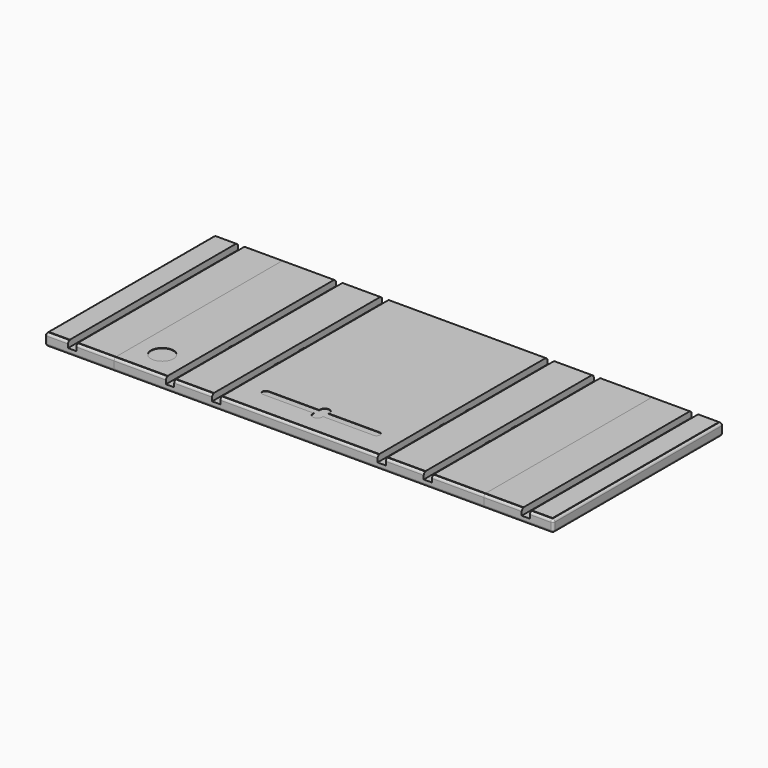
from build123d import *

# Parameters (mm, degrees)
F0_W         = 800
F0_H         = 460
F1_DEPTH     = 25
F2_R         = 5
F3_W         = 18
F3_H         = 13
F4_DEPTH     = 250
F6_DEPTH     = 25
F7_R         = 5
F7_2_R       = 5
F8_W         = 18
F8_H         = 13
F9_DEPTH     = 250
F10_W        = 150
F10_H        = 24
F11_DEPTH    = 30
F13_DEPTH    = 300
F14_R        = 20
F15_T1_DEPTH = 9
F16_R        = 5
F17_W        = 45
F17_H        = 450
F18_DEPTH    = 1
F17_W_2      = 82
F17_W_3      = 340
F19_DEPTH    = 1
F20_W        = 10
F20_H        = 15
F21_DEPTH    = 1
F22_R        = 24.5
F23_DEPTH    = 1


# Not quite as in the source:
# - a fillet or chamfer that OpenCascade refuses, or shapes differently, is made with other operations: its cross-section is extruded or revolved along the edge and cut away or added


with BuildPart() as f1:
    # F0 (on Top) → F1 (new body)
    with BuildSketch(Plane.XY):
        Rectangle(F0_W, F0_H)
    extrude(amount=F1_DEPTH)

    # F2
    f2_edges = [f1.edges().sort_by_distance(p)[0] for p in [
        (0, -230, 25),
        (0, 230, 25),
        (0, 230, 0),
        (0, -230, 0),
    ]]
    fillet(f2_edges, radius=F2_R)

    # F3 (on Front) → F4 (cut, symmetric)
    with BuildSketch(Plane.XZ):
        with Locations((-179, 18.5)):
            Rectangle(F3_W, F3_H)
        with Locations((-279, 18.5)):
            Rectangle(F3_W, F3_H)
        with Locations((179, 18.5)):
            Rectangle(F3_W, F3_H)
        with Locations((279, 18.5)):
            Rectangle(F3_W, F3_H)
    extrude(amount=F4_DEPTH, both=True, mode=Mode.SUBTRACT)

    # F10 (on Right) → F11 (cut, symmetric)
    with BuildSketch(Plane.YZ):
        with Locations((-11.93539612, 0)):
            Rectangle(F10_W, F10_H)
    extrude(amount=F11_DEPTH, both=True, mode=Mode.SUBTRACT)

    # F12 (on Right) → F13 (cut, symmetric)
    with BuildSketch(Plane.YZ):
        Polygon((-61.0856295228, 0), (-52.0856295228, 0), (-52.0856295228, 3), (-50.5856295228, 3), (-50.5856295228, 13), (-62.5856295228, 13), (-62.5856295228, 3), (-61.0856295228, 3), align=None)
        Polygon((6.4143704772, 3), (7.9143704772, 3), (7.9143704772, 0), (16.9143704772, 0), (16.9143704772, 3), (18.4143704772, 3), (18.4143704772, 13), (6.4143704772, 13), align=None)
    extrude(amount=F13_DEPTH, both=True, mode=Mode.SUBTRACT)

    # F14
    f14_edges = [f1.edges().sort_by_distance(p)[0] for p in [
        (30, -86.935396, 6),
        (-30, -86.935396, 6),
        (-30, 63.064604, 6),
        (30, 63.064604, 6),
    ]]
    fillet(f14_edges, radius=F14_R)

    # F15: fillet of radius 5 on 8 edges, made by hand

    # F15_s2 → F15_t1 (cut)
    with BuildSketch(Plane.XY.offset(3)):
        with BuildLine():
            ThreePointArc((-29.9932339999, -67.4555828422), (-31.5022899583, -64.0044123133), (-34.9915424999, -62.5856295228))
            Line((-34.9915424999, -62.5856295228), (-34.9915424999, -62.0856295228))
            Line((-34.9915424999, -62.0856295228), (-30, -62.0856295228))
            Line((-30, -62.0856295228), (-29.5, -62.5856295228))
            ThreePointArc((-29.5, -62.5856295228), (-29.5, -66.93539612), (-29.4934031499, -67.4425781742))
            Line((-29.4934031499, -67.4425781742), (-29.9932339999, -67.4555828422))
        make_face()
        with BuildLine():
            ThreePointArc((-30, -45.5856295228), (-31.4644660941, -49.1211634287), (-35, -50.5856295228))
            Line((-35, -50.5856295228), (-30, -50.5856295228))
            Line((-30, -50.5856295228), (-30, -45.5856295228))
        make_face()
        with BuildLine():
            ThreePointArc((-30, 1.4143704772), (-31.4644660941, 4.9499043831), (-35, 6.4143704772))
            Line((-35, 6.4143704772), (-30, 6.4143704772))
            Line((-30, 6.4143704772), (-30, 1.4143704772))
        make_face()
        with BuildLine():
            ThreePointArc((-30, 23.4143704772), (-31.4644660941, 19.8788365713), (-35, 18.4143704772))
            Line((-35, 18.4143704772), (-30, 18.4143704772))
            Line((-30, 18.4143704772), (-30, 23.4143704772))
        make_face()
        with BuildLine():
            ThreePointArc((29.9932339999, -67.4555828422), (31.5022899583, -64.0044123133), (34.9915424999, -62.5856295228))
            Line((34.9915424999, -62.5856295228), (34.9915424999, -62.0856295228))
            Line((34.9915424999, -62.0856295228), (30, -62.0856295228))
            Line((30, -62.0856295228), (29.5, -62.5856295228))
            ThreePointArc((29.5, -62.5856295228), (29.5, -66.93539612), (29.4934031499, -67.4425781742))
            Line((29.4934031499, -67.4425781742), (29.9932339999, -67.4555828422))
        make_face()
        with BuildLine():
            ThreePointArc((30, -45.5856295228), (31.4644660941, -49.1211634287), (35, -50.5856295228))
            Line((35, -50.5856295228), (30, -50.5856295228))
            Line((30, -50.5856295228), (30, -45.5856295228))
        make_face()
        with BuildLine():
            ThreePointArc((30, 1.4143704772), (31.4644660941, 4.9499043831), (35, 6.4143704772))
            Line((35, 6.4143704772), (30, 6.4143704772))
            Line((30, 6.4143704772), (30, 1.4143704772))
        make_face()
        with BuildLine():
            ThreePointArc((30, 23.4143704772), (31.4644660941, 19.8788365713), (35, 18.4143704772))
            Line((35, 18.4143704772), (30, 18.4143704772))
            Line((30, 18.4143704772), (30, 23.4143704772))
        make_face()
    extrude(amount=F15_T1_DEPTH, mode=Mode.SUBTRACT)

    # F16
    f16_edges = [f1.edges().sort_by_distance(p)[0] for p in [
        (-30, -61.08563, 1.5),
        (-30, -52.08563, 1.5),
        (-30, 7.91437, 1.5),
        (-30, 16.91437, 1.5),
        (30, 16.91437, 1.5),
        (30, 7.91437, 1.5),
        (30, -52.08563, 1.5),
        (30, -61.08563, 1.5),
    ]]
    fillet(f16_edges, radius=F16_R)


with BuildPart() as f6:
    # F5 (on Top) → F6 (new body)
    with BuildSketch(Plane.XY):
        Polygon((-400, -230), (-400, 0), (-400, 230), (-550, 230), (-550, -230), align=None)
    extrude(amount=F6_DEPTH)

    # F7
    f7_edges = [f6.edges().sort_by_distance(p)[0] for p in [
        (-475, 230, 25),
        (-550, 0, 25),
        (-475, -230, 25),
        (-475, -230, 0),
        (-550, 0, 0),
        (-475, 230, 0),
        (-550, -230, 12.5),
        (-550, 230, 12.5),
    ]]
    fillet(f7_edges, radius=F7_R)


with BuildPart() as f6b:
    # F5 (on Top) → F6, piece 2 (new body)
    with BuildSketch(Plane.XY):
        Polygon((400, 0), (400, -230), (550, -230), (550, 230), (400, 230), align=None)
    extrude(amount=F6_DEPTH)

    # F7#2
    f7_2_edges = [f6b.edges().sort_by_distance(p)[0] for p in [
        (475, 230, 0),
        (550, 0, 0),
        (475, -230, 0),
        (475, 230, 25),
        (475, -230, 25),
        (550, 0, 25),
        (550, -230, 12.5),
        (550, 230, 12.5),
    ]]
    fillet(f7_2_edges, radius=F7_2_R)


with BuildPart() as f9_tool:
    # F8 (on Front) → F9 (new body, symmetric)
    with BuildSketch(Plane.XZ):
        with Locations((-491, 18.5)):
            Rectangle(F8_W, F8_H)
        with Locations((491, 18.5)):
            Rectangle(F8_W, F8_H)
    extrude(amount=F9_DEPTH, both=True)


with BuildPart() as f6_1:
    add(f6.part)

    # F9: cut by f9_tool
    add(f9_tool.part, mode=Mode.SUBTRACT)


with BuildPart() as f6b_1:
    add(f6b.part)

    # F9: cut by f9_tool
    add(f9_tool.part, mode=Mode.SUBTRACT)


with BuildPart() as f18:
    # F17 (on face) → F18 (new body)
    with BuildSketch(Plane.XY.offset(25)):
        with Locations((-522.5, 0)):
            Rectangle(F17_W, F17_H)
    extrude(amount=F18_DEPTH)


with BuildPart() as f18b:
    # F17 (on face) → F18, piece 2 (new body)
    with BuildSketch(Plane.XY.offset(25)):
        with Locations((-441, 0)):
            Rectangle(F17_W_2, F17_H)
    extrude(amount=F18_DEPTH)


with BuildPart() as f18c:
    # F17 (on face) → F18, piece 3 (new body)
    with BuildSketch(Plane.XY.offset(25)):
        with Locations((-229, 0)):
            Rectangle(F17_W_2, F17_H)
    extrude(amount=F18_DEPTH)


with BuildPart() as f18d:
    # F17 (on face) → F18, piece 4 (new body)
    with BuildSketch(Plane.XY.offset(25)):
        Rectangle(F17_W_3, F17_H)
    extrude(amount=F18_DEPTH)

    # F20 (on face) → F21 (cut)
    with BuildSketch(Plane.XY.offset(26)):
        with BuildLine():
            ThreePointArc((-120, -162.5), (-127.5, -170), (-120, -177.5))
            Line((-120, -177.5), (-10, -177.5))
            Line((-10, -177.5), (-10, -162.5))
            Line((-10, -162.5), (-120, -162.5))
        make_face()
        with Locations((-5, -170)):
            Rectangle(F20_W, F20_H)
        with BuildLine():
            Line((0, -177.5), (-10, -177.5))
            Line((-10, -177.5), (-10, -180))
            ThreePointArc((-10, -180), (0, -190), (10, -180))
            Line((10, -180), (10, -177.5))
            Line((10, -177.5), (0, -177.5))
        make_face()
        with BuildLine():
            Line((-10, -160), (-10, -162.5))
            Line((-10, -162.5), (0, -162.5))
            Line((0, -162.5), (10, -162.5))
            Line((10, -162.5), (10, -160))
            ThreePointArc((10, -160), (0, -150), (-10, -160))
        make_face()
        with Locations((5, -170)):
            Rectangle(F20_W, F20_H)
        with BuildLine():
            Line((10, -162.5), (10, -177.5))
            Line((10, -177.5), (120, -177.5))
            ThreePointArc((120, -177.5), (127.5, -170), (120, -162.5))
            Line((120, -162.5), (10, -162.5))
        make_face()
    extrude(amount=-F21_DEPTH, mode=Mode.SUBTRACT)


with BuildPart() as f18e:
    # F17 (on face) → F18, piece 5 (new body)
    with BuildSketch(Plane.XY.offset(25)):
        with Locations((229, 0)):
            Rectangle(F17_W_2, F17_H)
    extrude(amount=F18_DEPTH)


with BuildPart() as f18f:
    # F17 (on face) → F18, piece 6 (new body)
    with BuildSketch(Plane.XY.offset(25)):
        with Locations((441, 0)):
            Rectangle(F17_W_2, F17_H)
    extrude(amount=F18_DEPTH)


with BuildPart() as f18g:
    # F17 (on face) → F18, piece 7 (new body)
    with BuildSketch(Plane.XY.offset(25)):
        with Locations((522.5, 0)):
            Rectangle(F17_W, F17_H)
    extrude(amount=F18_DEPTH)


with BuildPart() as f19:
    # F19 (new): a face of the model
    f19_faces = [f1.part.faces().sort_by_distance(p)[0] for p in [
        (-344, 0, 25),
    ]]
    extrude(f19_faces, amount=F19_DEPTH)

    # F22 (on face) → F23 (cut)
    with BuildSketch(Plane.XY.offset(26)):
        with Locations((-344, -170)):
            Circle(F22_R)
    extrude(amount=-F23_DEPTH, mode=Mode.SUBTRACT)


with BuildPart() as f19b:
    # F19#2 (new): a face of the model
    f19_2_faces = [f1.part.faces().sort_by_distance(p)[0] for p in [
        (344, 0, 25),
    ]]
    extrude(f19_2_faces, amount=F19_DEPTH)


solid = Compound([f1.part, f6_1.part, f6b_1.part, f18.part, f18b.part, f18c.part, f18d.part, f18e.part, f18f.part, f18g.part, f19.part, f19b.part])
